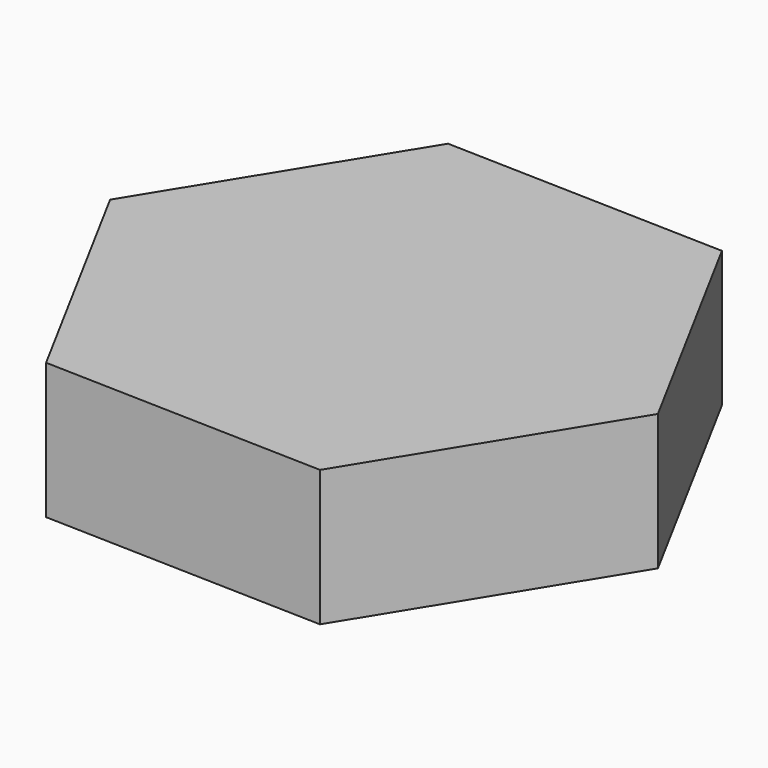
from build123d import *

# Parameters (mm, degrees)
F3_DEPTH = 25.4


# Not quite as in the source:
# - the program builds the solid bodies; features that only make, move or delete a surface that nothing else refers to are left out


with BuildPart() as f3:
    # F2 (on face) → F3 (new body)
    with BuildSketch(Plane.XY):
        Polygon((-91.0365809017, 103.5870710301), (-118.4836845583, 58.9960863901), (-93.5903109086, 12.9307050432), (-41.2498336023, 11.4563083363), (-13.8027299458, 56.0472929763), (-38.6961035955, 102.1126743232), align=None)
    extrude(amount=F3_DEPTH)


solid = f3.part
